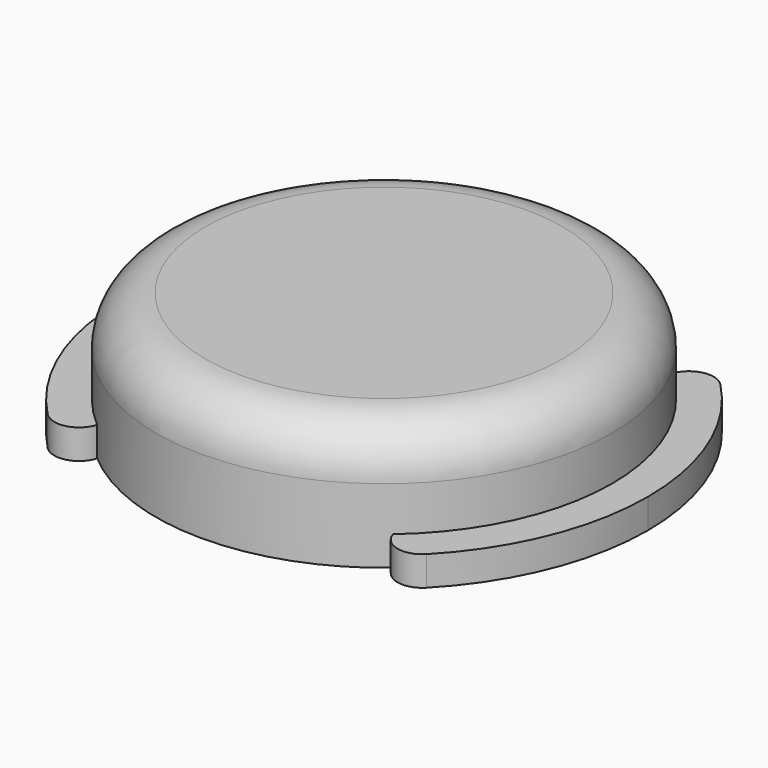
from build123d import *

# Parameters (mm, degrees)
F0_R        = 9.25
F1_DEPTH    = 5
F3_DEPTH    = 1.2
F4_T1_DEPTH = 12.1393431135
F5_R        = 2


# Not quite as in the source:
# - a fillet or chamfer that OpenCascade refuses, or shapes differently, is made with other operations: its cross-section is extruded or revolved along the edge and cut away or added


with BuildPart() as f1:
    # F0 (on Top) → F1 (new body)
    with BuildSketch(Plane.XY):
        Circle(F0_R)
    extrude(amount=F1_DEPTH)

    # F2 (on face) → F3 (join)
    with BuildSketch(Plane(origin=(0, 0, 0), x_dir=(1, 0, 0), z_dir=(0, 0, -1))):
        with BuildLine():
            Line((-6, 7.0400639202), (-6, 8.8594582227))
            ThreePointArc((-6, 8.8594582227), (-10.7, 0), (-6, -8.8594582227))
            Line((-6, -8.8594582227), (-6, -7.0400639202))
            ThreePointArc((-6, -7.0400639202), (-9.25, 0), (-6, 7.0400639202))
        make_face()
        with BuildLine():
            Line((-6, -7.0400639202), (-6, 7.0400639202))
            ThreePointArc((-6, 7.0400639202), (-9.25, 0), (-6, -7.0400639202))
        make_face()
        with BuildLine():
            Line((6, -7.0400639202), (6, 7.0400639202))
            ThreePointArc((6, 7.0400639202), (0, 9.25), (-6, 7.0400639202))
            Line((-6, 7.0400639202), (-6, -7.0400639202))
            ThreePointArc((-6, -7.0400639202), (0, -9.25), (6, -7.0400639202))
        make_face()
        with BuildLine():
            ThreePointArc((9.25, 0), (8.3982885161, 3.8770156048), (6, 7.0400639202))
            Line((6, 7.0400639202), (6, -7.0400639202))
            ThreePointArc((6, -7.0400639202), (8.3982885161, -3.8770156048), (9.25, 0))
        make_face()
        with BuildLine():
            ThreePointArc((6, -8.8594582227), (9.4522484098, -5.0144790358), (10.7, 0))
            ThreePointArc((10.7, 0), (9.4522484098, 5.0144790358), (6, 8.8594582227))
            Line((6, 8.8594582227), (6, 7.0400639202))
            ThreePointArc((6, 7.0400639202), (8.3982885161, 3.8770156048), (9.25, 0))
            ThreePointArc((9.25, 0), (8.3982885161, -3.8770156048), (6, -7.0400639202))
            Line((6, -7.0400639202), (6, -8.8594582227))
        make_face()
    extrude(amount=-F3_DEPTH)

    # F4: fillet of radius 1 on 4 edges, made by hand

    # F4_s2 → F4_t1 (cut)
    with BuildSketch(Plane.XY.offset(-5.4696715568)):
        with BuildLine():
            ThreePointArc((6, -7.0400639202), (6.7195608847, -7.728089766), (7.6766055002, -7.4538398154))
            ThreePointArc((7.6766055002, -7.4538398154), (6.8743236234, -8.1996143032), (6, -8.8594582227))
            Line((6, -8.8594582227), (6, -7.0400639202))
        make_face()
        with BuildLine():
            ThreePointArc((-7.6766055002, -7.4538398154), (-6.7195608847, -7.728089766), (-6, -7.0400639202))
            Line((-6, -7.0400639202), (-6, -8.8594582227))
            ThreePointArc((-6, -8.8594582227), (-6.8743236234, -8.1996143032), (-7.6766055002, -7.4538398154))
        make_face()
        with BuildLine():
            ThreePointArc((7.6766055002, 7.4538398154), (6.7195608847, 7.728089766), (6, 7.0400639202))
            Line((6, 7.0400639202), (6, 8.8594582227))
            ThreePointArc((6, 8.8594582227), (6.8743236234, 8.1996143032), (7.6766055002, 7.4538398154))
        make_face()
        with BuildLine():
            ThreePointArc((-6, 7.0400639202), (-6.7195608847, 7.728089766), (-7.6766055002, 7.4538398154))
            ThreePointArc((-7.6766055002, 7.4538398154), (-6.8743236234, 8.1996143032), (-6, 8.8594582227))
            Line((-6, 8.8594582227), (-6, 7.0400639202))
        make_face()
    extrude(amount=F4_T1_DEPTH, mode=Mode.SUBTRACT)

    # F5
    f5_edges = [f1.edges().sort_by_distance(p)[0] for p in [
        (-9.25, 0, 5),
    ]]
    fillet(f5_edges, radius=F5_R)


solid = f1.part
